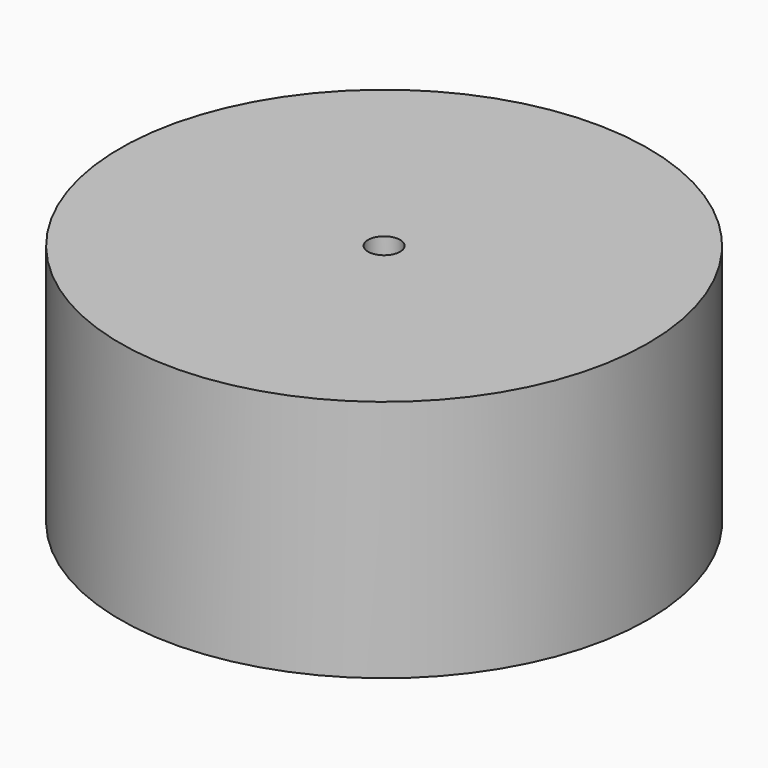
from build123d import *

# Parameters (mm, degrees)
F0_R     = 29.21
F1_DEPTH = 13.462
F2_R     = 1.778
F3_DEPTH = 2.54


# Not quite as in the source:
# - a pattern or mirror of a feature is missing from the dataset's text; its kind, count and spacing are read off the source's solid


with BuildPart() as f1:
    # F0 (on Top) → F1 (new body, symmetric)
    with BuildSketch(Plane.XY):
        Circle(F0_R)
    extrude(amount=F1_DEPTH, both=True)

    # F2 (on face) → F3 (cut)
    with BuildSketch(Plane.XY.offset(13.462)):
        Circle(F2_R)
    f3 = extrude(amount=-F3_DEPTH, mode=Mode.SUBTRACT)

    # F3_copies: F3 across plane
    add(f3.mirror(Plane(origin=(0, 0, 0), x_dir=(-1, 0, 0), z_dir=(0, 0, -1))), mode=Mode.SUBTRACT)


solid = f1.part
